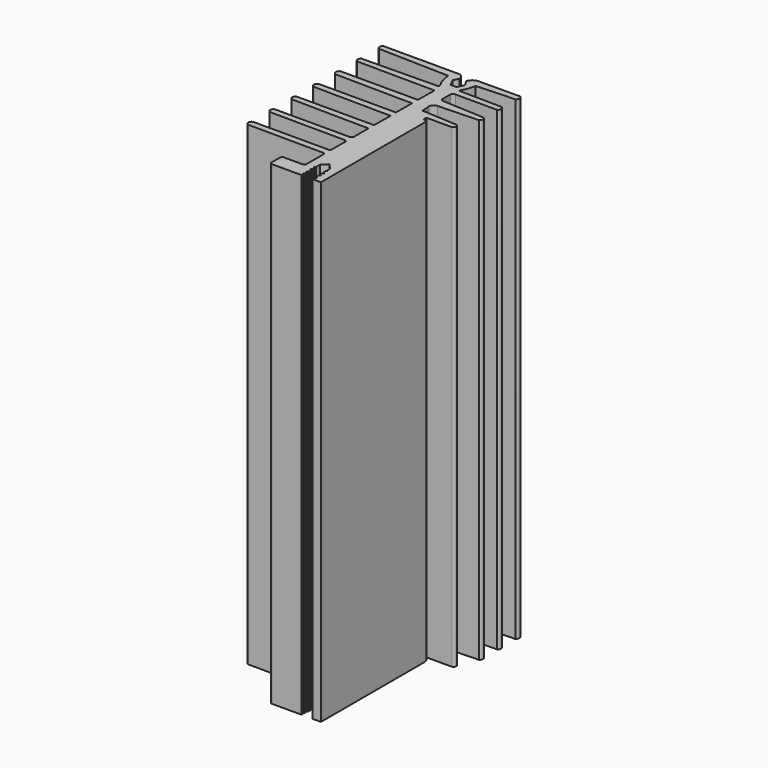
from build123d import *

# Parameters (mm, degrees)
F1_DEPTH      = 50.8
F1_DEPTH_BACK = 50.8


# Not quite as in the source:
# - a feature of the source that left no trace in its solid (it failed there, or was rolled back) is left out
# - the program builds the solid bodies; features that only make, move or delete a surface that nothing else refers to are left out


with BuildPart() as f1:
    # F0 (on Top) → F1 (new body, two sides)
    with BuildSketch(Plane.XY) as f1_sk:
        with BuildLine():
            Line((-3.3736736514, 24.7951317579), (-19.627969712, 24.8093213886))
            ThreePointArc((-19.627969712, 24.8093213886), (-20.0021253233, 24.2030567982), (-19.6617264301, 23.57721515))
            Line((-19.6617264301, 23.57721515), (-4.5088279332, 23.1754036615))
            ThreePointArc((-4.5088279332, 23.1754036615), (-4.1624050394, 21.325828975), (-3.3758739325, 19.6163541549))
            Line((-3.3758739325, 19.6163541549), (-3.3873883076, 19.2034132779))
            Line((-3.3873883076, 19.2034132779), (-19.6617264301, 18.969476223))
            ThreePointArc((-19.6617264301, 18.969476223), (-20.0032717352, 18.3534221724), (-19.6617264301, 17.7373681217))
            Line((-19.6617264301, 17.7373681217), (-2.9635052222, 17.5993758319))
            Line((-2.9635052222, 17.5993758319), (-3.0178399757, 13.2140200585))
            Line((-3.0178399757, 13.2140200585), (-19.4929447025, 13.2140200585))
            ThreePointArc((-19.4929447025, 13.2140200585), (-20.0233587748, 12.5220152549), (-19.4929447025, 11.8300104514))
            Line((-19.4929447025, 11.8300104514), (-3.0178399757, 11.6258831695))
            Line((-3.0178399757, 11.6258831695), (-3.0178399757, 7.360490039))
            Line((-3.0178399757, 7.360490039), (-19.4929447025, 7.360490039))
            ThreePointArc((-19.4929447025, 7.360490039), (-20.0219986391, 6.7022417206), (-19.4929447025, 6.0439934023))
            Line((-19.4929447025, 6.0439934023), (-2.9621112743, 5.8546986264))
            Line((-2.9621112743, 5.8546986264), (-3.0178399757, 1.493252581))
            Line((-3.0178399757, 1.493252581), (-19.4929447025, 1.493252581))
            ThreePointArc((-19.4929447025, 1.493252581), (-19.999079636, 0.8518822287), (-19.4929447025, 0.2105118765))
            Line((-19.4929447025, 0.2105118765), (-3.0178399757, 0))
            Line((-3.0178399757, 0), (-3.0178399757, -3.950452432))
            Line((-3.0178399757, -3.950452432), (-3.3726599067, -4.3803495355))
            Line((-3.3726599067, -4.3803495355), (-19.4929447025, -4.3803495355))
            ThreePointArc((-19.4929447025, -4.3803495355), (-20.0026487971, -5.0217199605), (-19.4929447025, -5.6630903855))
            Line((-19.4929447025, -5.6630903855), (-3.3726599067, -5.7729091495))
            Line((-3.3726599067, -5.7729091495), (-3.0178399757, -6.1277290806))
            Line((-3.0178399757, -6.1277290806), (-3.0178399757, -9.7752762958))
            Line((-3.0178399757, -9.7752762958), (-3.2525765998, -10.18643938))
            Line((-3.2525765998, -10.18643938), (-19.4929447025, -10.18643938))
            ThreePointArc((-19.4929447025, -10.18643938), (-20.0181876942, -10.8531266451), (-19.4929447025, -11.5198139101))
            Line((-19.4929447025, -11.5198139101), (-3.2525765998, -11.6145808049))
            Line((-3.2525765998, -11.6145808049), (-3.0190503156, -11.9383819401))
            Line((-3.0190503156, -11.9383819401), (-3.0190503156, -16.7704734888))
            Line((-3.0190503156, -16.7704734888), (-3.3736736514, -17.0262288302))
            Line((-3.3736736514, -17.0262288302), (-7.4309431948, -17.0262288302))
            ThreePointArc((-7.4309431948, -17.0262288302), (-7.7883055211, -17.1251856492), (-7.9560680315, -17.4558758736))
            Line((-7.9560680315, -17.4558758736), (-7.9560680315, -19.7419915348))
            ThreePointArc((-7.9560680315, -19.7419915348), (-7.8385182356, -20.0781647595), (-7.497502665, -20.1808232814))
            Line((-7.497502665, -20.1808232814), (-1.1584198955, -20.1714233881))
            Line((-1.1584198955, -20.1714233881), (-1.138712159, -19.8357657809))
            Line((-1.138712159, -19.8357657809), (-1.4197152341, -19.5692516863))
            Line((-1.4197152341, -19.5692516863), (-1.160888255, -19.2963536351))
            Line((-1.160888255, -19.2963536351), (-1.138712159, -18.9265421938))
            Line((-1.138712159, -18.9265421938), (-1.3017905422, -18.7004221842))
            Line((-1.3017905422, -18.7004221842), (-1.0179714863, -18.4957310875))
            Line((-1.0179714863, -18.4957310875), (-1.018282466, -17.9434493202))
            Line((-1.018282466, -17.9434493202), (-1.4397868638, -17.7126266085))
            Line((-1.4397868638, -17.7126266085), (-1.138712159, -17.3513367812))
            Line((-1.138712159, -17.3513367812), (-1.138712159, -16.8896894959))
            Line((-1.138712159, -16.8896894959), (-1.4169517005, -16.588565616))
            Line((-1.4169517005, -16.588565616), (-1.138712159, -16.3878984806))
            Line((-1.138712159, -16.3878984806), (-1.138712159, -15.3241008577))
            Line((-1.138712159, -15.3241008577), (0, -14.1900535673))
            Line((0, -14.1900535673), (1.0927112374, -15.4159043089))
            Line((1.0927112374, -15.4159043089), (1.1339221451, -16.1570739001))
            Line((1.1339221451, -16.1570739001), (1.3667184391, -16.3108690956))
            Line((1.3667184391, -16.3108690956), (1.0229069001, -16.558826939))
            Line((1.0229069001, -16.558826939), (1.0490959976, -17.0602984726))
            Line((1.0490959976, -17.0602984726), (1.462081531, -17.337922364))
            Line((1.462081531, -17.337922364), (1.1371706318, -17.572249013))
            Line((1.1371706318, -17.572249013), (1.1339221451, -18.033772707))
            Line((1.1339221451, -18.033772707), (1.4404929399, -18.274631373))
            Line((1.4404929399, -18.274631373), (1.1339221451, -18.4957310875))
            Line((1.1339221451, -18.4957310875), (1.1293826392, -19.1477481276))
            Line((1.1293826392, -19.1477481276), (1.5007078182, -19.3585008383))
            Line((1.5007078182, -19.3585008383), (1.1495453005, -19.6058004949))
            Line((1.1495453005, -19.6058004949), (1.1458612277, -20.178947635))
            Line((1.1458612277, -20.178947635), (2.9662006887, -20.178947635))
            Line((2.9662006887, -20.178947635), (2.9662006887, 7.7263202994))
            Line((2.9662006887, 7.7263202994), (2.825798234, 8.2537010312))
            Line((2.825798234, 8.2537010312), (2.1506715566, 8.2537010312))
            Line((2.1506715566, 8.2537010312), (2.1506715566, 9.0581281111))
            Line((2.1506715566, 9.0581281111), (7.5833620504, 9.0581281111))
            ThreePointArc((7.5833620504, 9.0581281111), (8.0257459726, 9.6480058962), (7.5632906519, 10.222283192))
            Line((7.5632906519, 10.222283192), (0.0440248574, 10.6278444304))
            Line((0.0440248574, 10.6278444304), (0, 11.1270683113))
            Line((0, 11.1270683113), (-0.1044616438, 12.3116206378))
            ThreePointArc((-0.1044616438, 12.3116206378), (0.126172228, 13.1274286151), (0.8690126706, 13.5359903798))
            Line((0.8690126706, 13.5359903798), (9.5102395862, 13.8351768255))
            ThreePointArc((9.5102395862, 13.8351768255), (9.9020840969, 14.4295718757), (9.570454247, 15.0595474616))
            Line((9.570454247, 15.0595474616), (0.6003075975, 15.5130466074))
            ThreePointArc((0.6003075975, 15.5130466074), (0.2149232739, 15.60577238), (0, 15.9388296306))
            Line((0, 15.9388296306), (0, 18.1245207787))
            ThreePointArc((0, 18.1245207787), (0.2171557282, 18.5044688755), (0.6286933785, 18.6533108354))
            Line((0.6286933785, 18.6533108354), (9.570454247, 18.6533108354))
            ThreePointArc((9.570454247, 18.6533108354), (9.9234885577, 19.2956030182), (9.570454247, 19.9378952011))
            Line((9.570454247, 19.9378952011), (0.3673353055, 20.0769044086))
            Line((0.3673353055, 20.0769044086), (0.3164518273, 20.2818233147))
            ThreePointArc((0.3164518273, 20.2818233147), (0.9977498793, 21.6728398839), (1.3667184391, 23.1771524623))
            Line((1.3667184391, 23.1771524623), (9.570454247, 23.5285814479))
            ThreePointArc((9.570454247, 23.5285814479), (9.9232117791, 24.1969227418), (9.570454247, 24.8652640357))
            Line((9.570454247, 24.8652640357), (0.5151510704, 24.7951317579))
            ThreePointArc((0.5151510704, 24.7951317579), (-0.4052105617, 24.3861366082), (-0.9608993423, 23.5461648554))
            Line((-0.9608993423, 23.5461648554), (-0.1758071594, 22.2885161638))
            Line((-0.1758071594, 22.2885161638), (-0.8712234916, 20.8444888061))
            Line((-0.8712234916, 20.8444888061), (-2.148604719, 20.8550449461))
            Line((-2.148604719, 20.8550449461), (-2.9008225538, 22.3878659308))
            Line((-2.9008225538, 22.3878659308), (-2.3517927621, 23.5461648554))
            ThreePointArc((-2.3517927621, 23.5461648554), (-2.6533703145, 24.3419450304), (-3.3736736514, 24.7951317579))
        make_face()
    extrude(amount=F1_DEPTH)
    extrude(f1_sk.sketch, amount=-F1_DEPTH_BACK)


solid = f1.part
